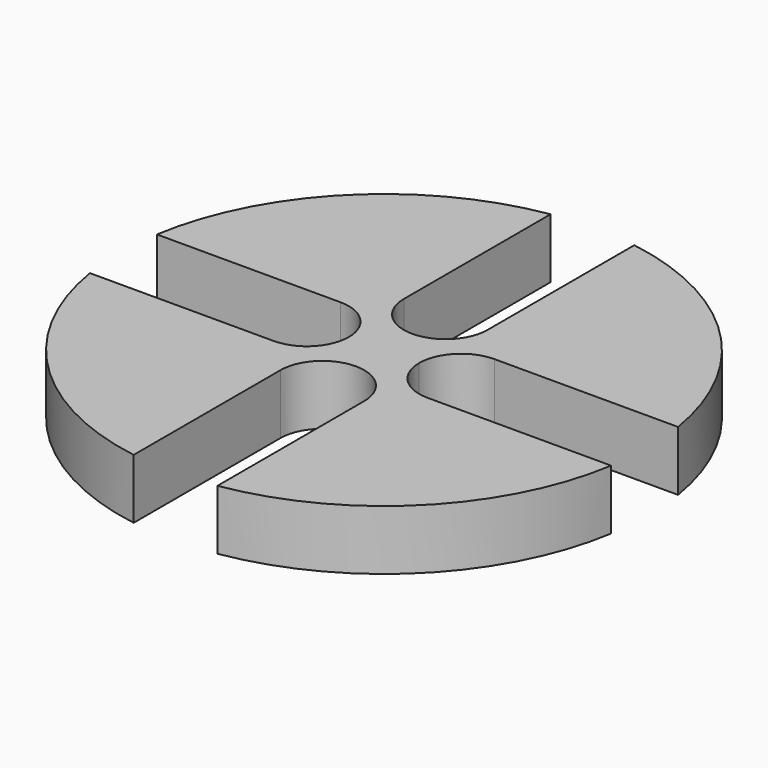
from build123d import *

# Parameters (mm, degrees)
F1_DEPTH = 17


# Not quite as in the source:
# - a feature of the source that left no trace in its solid (it failed there, or was rolled back) is left out


with BuildPart() as f1:
    # F0 (on Top) → F1 (new body)
    with BuildSketch(Plane.XY):
        with BuildLine():
            Line((21.9, 11.9), (74.0499155975, 11.9))
            ThreePointArc((74.0499155975, 11.9), (53.033008589, 53.033008589), (11.9, 74.0499155975))
            Line((11.9, 74.0499155975), (11.9, 21.9))
            ThreePointArc((11.9, 21.9), (0, 10), (-11.9, 21.9))
            Line((-11.9, 21.9), (-11.9, 74.0499155975))
            ThreePointArc((-11.9, 74.0499155975), (-53.033008589, 53.033008589), (-74.0499155975, 11.9))
            Line((-74.0499155975, 11.9), (-21.9, 11.9))
            ThreePointArc((-21.9, 11.9), (-10, 0), (-21.9, -11.9))
            Line((-21.9, -11.9), (-74.0499155975, -11.9))
            ThreePointArc((-74.0499155975, -11.9), (-53.033008589, -53.033008589), (-11.9, -74.0499155975))
            Line((-11.9, -74.0499155975), (-11.9, -21.9))
            ThreePointArc((-11.9, -21.9), (0, -10), (11.9, -21.9))
            Line((11.9, -21.9), (11.9, -74.0499155975))
            ThreePointArc((11.9, -74.0499155975), (53.033008589, -53.033008589), (74.0499155975, -11.9))
            Line((74.0499155975, -11.9), (21.9, -11.9))
            ThreePointArc((21.9, -11.9), (13.4854293039, -8.4145706961), (10, 0))
            ThreePointArc((10, 0), (13.4854293039, 8.4145706961), (21.9, 11.9))
        make_face()
    extrude(amount=F1_DEPTH)


solid = f1.part
